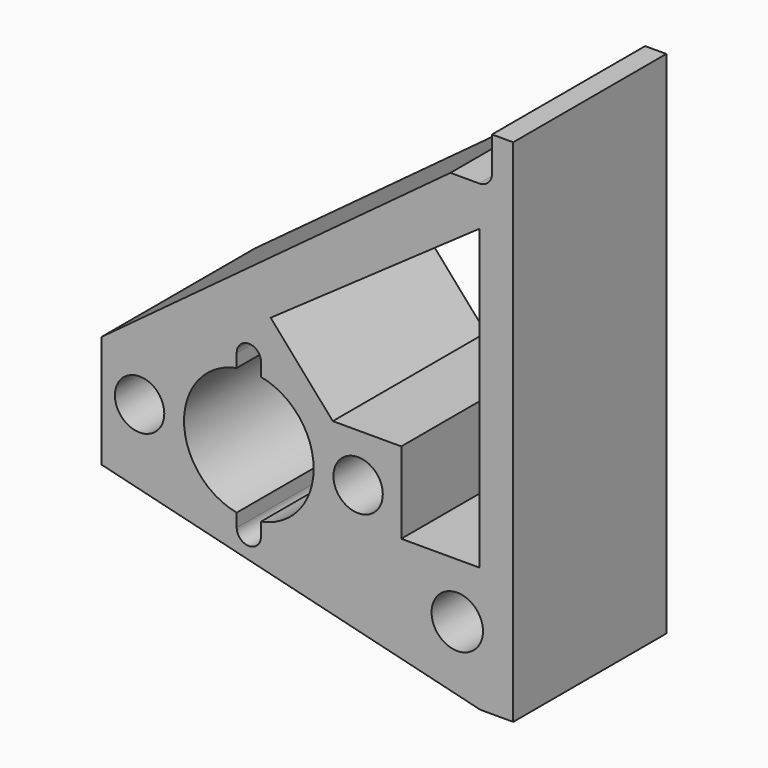
from build123d import *

# Parameters (mm, degrees)
F1_R     = 3.048
F1_R_2   = 3.175
F2_DEPTH = 11.811


# Not quite as in the source:
# - a variable given as a bare number and used for a length is read in inches; the dataset says mm whatever the document's units were


with BuildPart() as f2:
    # F1 (on Front) → F2 (new body, symmetric)
    with BuildSketch(Plane.XZ):
        with BuildLine():
            Line((-4.0742880665, 0), (0, 0))
            Line((0, 0), (0, 62.992))
            Line((0, 62.992), (-2.6162, 62.992))
            Line((-2.6162, 62.992), (-2.6162, 58.7375))
            ThreePointArc((-2.6162, 58.7375), (-3.0811679849, 57.6149679849), (-4.2037, 57.15))
            Line((-4.2037, 57.15), (-7.7502694912, 57.15))
            Line((-7.7502694912, 57.15), (-50.8, 25.3296804607))
            Line((-50.8, 25.3296804607), (-50.8, 11.4263528958))
            Line((-50.8, 11.4263528958), (-4.0742880665, 0))
        make_face()
        with Locations((-46.1220345246, 19.5037350059)):
            Circle(F1_R, mode=Mode.SUBTRACT)
        with BuildLine():
            ThreePointArc((-31.1360345246, 27.3631369577), (-26.4699650444, 24.6040145276), (-24.6336345246, 19.5037350059))
            ThreePointArc((-24.6336345246, 19.5037350059), (-26.4699650444, 14.4034554841), (-31.1360345246, 11.6443330541))
            Line((-31.1360345246, 11.6443330541), (-31.1360345246, 10.0041350059))
            ThreePointArc((-31.1360345246, 10.0041350059), (-32.6346345246, 8.5055350059), (-34.1332345246, 10.0041350059))
            Line((-34.1332345246, 10.0041350059), (-34.1332345246, 11.6443330541))
            ThreePointArc((-34.1332345246, 11.6443330541), (-40.6356345246, 19.5037350059), (-34.1332345246, 27.3631369577))
            Line((-34.1332345246, 27.3631369577), (-34.1332345246, 29.0033350059))
            ThreePointArc((-34.1332345246, 29.0033350059), (-32.6346345246, 30.5019350059), (-31.1360345246, 29.0033350059))
            Line((-31.1360345246, 29.0033350059), (-31.1360345246, 27.3631369577))
        make_face(mode=Mode.SUBTRACT)
        with Locations((-6.9088, 8.636)):
            Circle(F1_R_2, mode=Mode.SUBTRACT)
        with Locations((-19.1472345246, 19.5037350059)):
            Circle(F1_R, mode=Mode.SUBTRACT)
        Polygon((-29.9449488521, 34.1863036156), (-4.1464217938, 52.254665643), (-4.1464217938, 15.4098803177), (-13.8212321326, 15.4098803177), (-13.8212321326, 25.4460312426), (-22.2725905478, 25.4460312426), align=None, mode=Mode.SUBTRACT)
    extrude(amount=F2_DEPTH, both=True)


solid = f2.part
